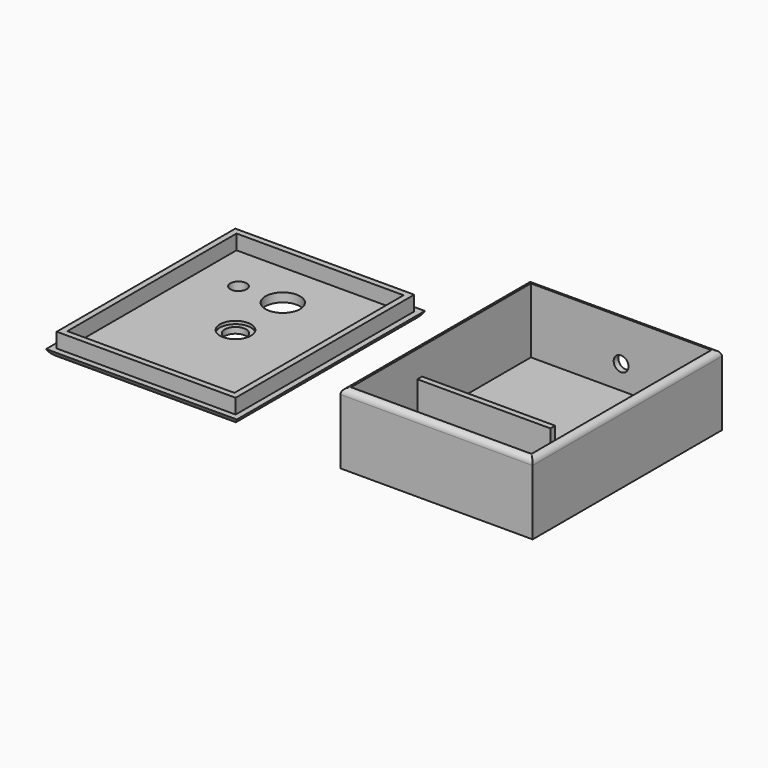
from build123d import *

# Parameters (mm, degrees)
F1_DEPTH     = 2
F0_W         = 65
F0_H         = 80
F2_DEPTH     = 24
F0_W_2       = 45
F0_H_2       = 2
F3_DEPTH     = 15
F4_R         = 2.5
F5_DEPTH     = 2
F6_R         = 1.99999
F0_W_3       = 64.5
F0_H_3       = 79.5
F0_W_4       = 60.5
F0_H_4       = 75.5
F7_DEPTH     = 3
F0_W_5       = 56.5
F0_H_5       = 71.5
F0_R         = 5.25
F0_R_2       = 2.75
F0_R_3       = 5.875
F8_DEPTH     = 8
F0_R_4       = 3.625
F9_DEPTH     = 2
F10_T1_DEPTH = 87.4128784748
F10_T3_DEPTH = 102.4128784748


# Not quite as in the source:
# - a fillet or chamfer that OpenCascade refuses, or shapes differently, is made with other operations: its cross-section is extruded or revolved along the edge and cut away or added
# - a fillet or chamfer is up to 0.001 mm smaller than in the source, because OpenCascade refuses the exact size


with BuildPart() as f1:
    # F0 (on Top) → F1 (new body)
    with BuildSketch(Plane.XY):
        Polygon((30.5, 38), (-30.5, 38), (-30.5, -8), (14.5, -8), (14.5, -10), (-30.5, -10), (-30.5, -38), (30.5, -38), align=None)
    extrude(amount=F1_DEPTH)

    # F0 (on Top) → F2 (join)
    with BuildSketch(Plane.XY):
        Rectangle(F0_W, F0_H)
        Polygon((-30.5, -8), (-30.5, 38), (30.5, 38), (30.5, -38), (-30.5, -38), (-30.5, -10), align=None, mode=Mode.SUBTRACT)
    extrude(amount=F2_DEPTH)

    # F0 (on Top) → F3 (join)
    with BuildSketch(Plane.XY):
        with Locations((-8, -9)):
            Rectangle(F0_W_2, F0_H_2)
    extrude(amount=F3_DEPTH)

    # F4 (on face) → F5 (cut, through all)
    with BuildSketch(Plane(origin=(0, 40, 0), x_dir=(-1, 0, 0), z_dir=(0, 1, 0))):
        with Locations((0, 10)):
            Circle(F4_R)
    extrude(amount=-F5_DEPTH, mode=Mode.SUBTRACT)

    # F6 (radius 2 in the source; OpenCascade refuses exactly that, so slightly less here)
    f6_edges = [f1.edges().sort_by_distance(p)[0] for p in [
        (-32.5, 0, 24),
        (0, 40, 24),
        (32.5, 0, 24),
        (0, -40, 24),
    ]]
    fillet(f6_edges, radius=F6_R)


with BuildPart() as f7:
    # F0 (on Top) → F7 (new body)
    with BuildSketch(Plane.XY):
        with Locations((-100, 0)):
            Rectangle(F0_W_3, F0_H_3)
        with Locations((-100, 0)):
            Rectangle(F0_W_4, F0_H_4, mode=Mode.SUBTRACT)
    extrude(amount=F7_DEPTH)



with BuildPart() as f7b:
    # F0 (on Top) → F7, piece 2 (new body)
    with BuildSketch(Plane.XY):
        with Locations((-100, 0)):
            Rectangle(F0_W_5, F0_H_5)
        with Locations((-100, 0)):
            Circle(F0_R, mode=Mode.SUBTRACT)
        with Locations((-115, 20)):
            Circle(F0_R_2, mode=Mode.SUBTRACT)
        with Locations((-100, 20)):
            Circle(F0_R_3, mode=Mode.SUBTRACT)
    extrude(amount=F7_DEPTH)


with BuildPart() as f7_1:
    add(f7.part)

    add(f7b.part)  # F8 merges F7b
    # F0 (on Top) → F8 (join)
    with BuildSketch(Plane.XY):
        with Locations((-100, 0)):
            Rectangle(F0_W_4, F0_H_4)
        with Locations((-100, 0)):
            Rectangle(F0_W_5, F0_H_5, mode=Mode.SUBTRACT)
    extrude(amount=F8_DEPTH)

    # F0 (on Top) → F9 (join)
    with BuildSketch(Plane.XY):
        with Locations((-100, 0)):
            Circle(F0_R)
        with Locations((-100, 0)):
            Circle(F0_R_4, mode=Mode.SUBTRACT)
    extrude(amount=F9_DEPTH)

    # F10: fillet of radius 5 on 4 edges, made by hand

    # F10_s2 → F10_t1 (cut)
    with BuildSketch(Plane.YZ.offset(-143.7064392374)):
        with BuildLine():
            ThreePointArc((35.167424305, 0), (37.9060370926, 0.8166998673), (39.75, 3))
            Line((39.75, 3), (39.75, 0))
            Line((39.75, 0), (35.167424305, 0))
        make_face()
        with BuildLine():
            ThreePointArc((-35.167424305, 0), (-37.9060370926, 0.8166998673), (-39.75, 3))
            Line((-39.75, 3), (-39.75, 0))
            Line((-39.75, 0), (-35.167424305, 0))
        make_face()
    extrude(amount=F10_T1_DEPTH, mode=Mode.SUBTRACT)

    # F10_s4 → F10_t3 (cut)
    with BuildSketch(Plane.XZ.offset(-51.2064392374)):
        with BuildLine():
            ThreePointArc((-127.667424305, 0), (-130.4060370926, 0.8166998673), (-132.25, 3))
            Line((-132.25, 3), (-132.25, 0))
            Line((-132.25, 0), (-127.667424305, 0))
        make_face()
        with BuildLine():
            ThreePointArc((-72.332575695, 0), (-69.5939629074, 0.8166998673), (-67.75, 3))
            Line((-67.75, 3), (-67.75, 0))
            Line((-67.75, 0), (-72.332575695, 0))
        make_face()
    extrude(amount=F10_T3_DEPTH, mode=Mode.SUBTRACT)


solid = Compound([f1.part, f7_1.part])
